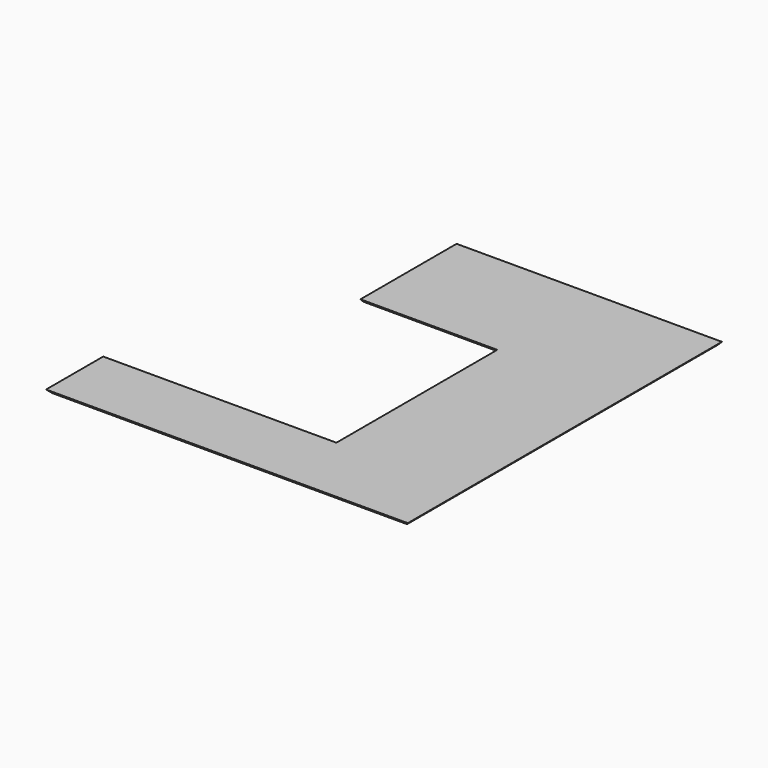
from build123d import *

# Parameters (mm, degrees)
F1_DEPTH = 19.05
F2_SIZE  = 19.04999


# Not quite as in the source:
# - a fillet or chamfer is up to 0.001 mm smaller than in the source, because OpenCascade refuses the exact size


with BuildPart() as f1:
    # F0 (on Top) → F1 (new body)
    with BuildSketch(Plane.XY):
        Polygon((1244.6, 0), (0, 0), (0, -381), (1930.4, -381), (1930.4, 1714.5), (514.35, 1714.5), (514.35, 1073.15), (1244.6, 1073.15), align=None)
    extrude(amount=F1_DEPTH)

    # F2 (size 19.05 in the source; OpenCascade refuses exactly that, so slightly less here)
    f2_edges = [f1.edges().sort_by_distance(p)[0] for p in [
        (965.2, -381, 0),
        (1930.4, 666.75, 0),
        (879.475, 1073.15, 0),
        (1244.6, 536.575, 0),
        (622.3, 0, 0),
        (0, -190.5, 0),
    ]]
    chamfer(f2_edges, length=F2_SIZE)


solid = f1.part
